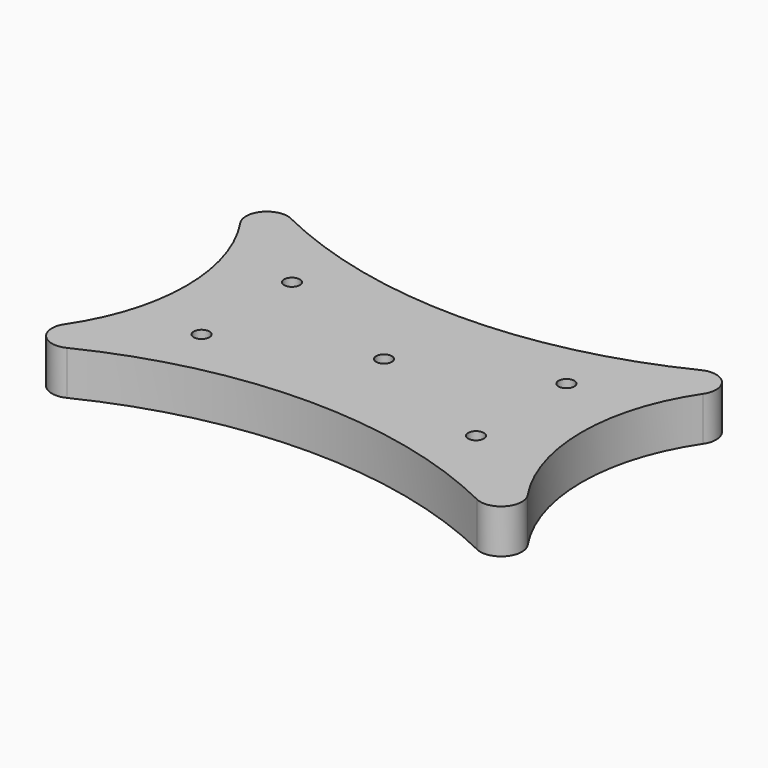
from build123d import *

# Parameters (mm, degrees)
F0_R     = 3.175
F1_DEPTH = 19.05
F2_DEPTH = 22.225
F3_DEPTH = 4.445


# Not quite as in the source:
# - a feature names something its author has since deleted; it is built from what else it names


with BuildPart() as f1:
    # F0 (on Top) → F1 (new body)
    with BuildSketch(Plane.XY):
        with BuildLine():
            ThreePointArc((82.8215071839, 56.5294814298), (0, 37.38), (-82.8215071839, 56.5294814298))
            ThreePointArc((-82.8215071839, 56.5294814298), (-92.8246316261, 54.4975844509), (-93.4439756283, 44.3089870526))
            ThreePointArc((-93.4439756283, 44.3089870526), (-79.88, 0), (-93.4439756283, -44.3089870526))
            ThreePointArc((-93.4439756283, -44.3089870526), (-92.8246316261, -54.4975844509), (-82.8215071839, -56.5294814298))
            ThreePointArc((-82.8215071839, -56.5294814298), (0, -37.38), (82.8215071839, -56.5294814298))
            ThreePointArc((82.8215071839, -56.5294814298), (92.8246316261, -54.4975844509), (93.4439756283, -44.3089870526))
            ThreePointArc((93.4439756283, -44.3089870526), (79.88, 0), (93.4439756283, 44.3089870526))
            ThreePointArc((93.4439756283, 44.3089870526), (92.8246316261, 54.4975844509), (82.8215071839, 56.5294814298))
        make_face()
        with Locations((-55.4007254541, -22.8000469506)):
            Circle(F0_R, mode=Mode.SUBTRACT)
        Circle(F0_R, mode=Mode.SUBTRACT)
        with Locations((55.4007254541, -22.8000469506)):
            Circle(F0_R, mode=Mode.SUBTRACT)
        with Locations((-55.4007254541, 22.8000469506)):
            Circle(F0_R, mode=Mode.SUBTRACT)
        with Locations((55.4007254541, 22.8000469506)):
            Circle(F0_R, mode=Mode.SUBTRACT)
    extrude(amount=F1_DEPTH)

    # F0 (on Top) → F2 (join)
    with BuildSketch(Plane.XY):
        with BuildLine():
            ThreePointArc((82.8215071839, 56.5294814298), (0, 37.38), (-82.8215071839, 56.5294814298))
            ThreePointArc((-82.8215071839, 56.5294814298), (-92.8246316261, 54.4975844509), (-93.4439756283, 44.3089870526))
            ThreePointArc((-93.4439756283, 44.3089870526), (-79.88, 0), (-93.4439756283, -44.3089870526))
            ThreePointArc((-93.4439756283, -44.3089870526), (-92.8246316261, -54.4975844509), (-82.8215071839, -56.5294814298))
            ThreePointArc((-82.8215071839, -56.5294814298), (0, -37.38), (82.8215071839, -56.5294814298))
            ThreePointArc((82.8215071839, -56.5294814298), (92.8246316261, -54.4975844509), (93.4439756283, -44.3089870526))
            ThreePointArc((93.4439756283, -44.3089870526), (79.88, 0), (93.4439756283, 44.3089870526))
            ThreePointArc((93.4439756283, 44.3089870526), (92.8246316261, 54.4975844509), (82.8215071839, 56.5294814298))
        make_face()
        with Locations((-55.4007254541, -22.8000469506)):
            Circle(F0_R, mode=Mode.SUBTRACT)
        Circle(F0_R, mode=Mode.SUBTRACT)
        with Locations((55.4007254541, -22.8000469506)):
            Circle(F0_R, mode=Mode.SUBTRACT)
        with Locations((-55.4007254541, 22.8000469506)):
            Circle(F0_R, mode=Mode.SUBTRACT)
        with Locations((55.4007254541, 22.8000469506)):
            Circle(F0_R, mode=Mode.SUBTRACT)
    extrude(amount=F2_DEPTH)

    # F0 (on Top) → F3 (cut)
    with BuildSketch(Plane.XY):
        with BuildLine():
            ThreePointArc((82.8215071839, 56.5294814298), (0, 37.38), (-82.8215071839, 56.5294814298))
            ThreePointArc((-82.8215071839, 56.5294814298), (-92.8246316261, 54.4975844509), (-93.4439756283, 44.3089870526))
            ThreePointArc((-93.4439756283, 44.3089870526), (-79.88, 0), (-93.4439756283, -44.3089870526))
            ThreePointArc((-93.4439756283, -44.3089870526), (-92.8246316261, -54.4975844509), (-82.8215071839, -56.5294814298))
            ThreePointArc((-82.8215071839, -56.5294814298), (0, -37.38), (82.8215071839, -56.5294814298))
            ThreePointArc((82.8215071839, -56.5294814298), (92.8246316261, -54.4975844509), (93.4439756283, -44.3089870526))
            ThreePointArc((93.4439756283, -44.3089870526), (79.88, 0), (93.4439756283, 44.3089870526))
            ThreePointArc((93.4439756283, 44.3089870526), (92.8246316261, 54.4975844509), (82.8215071839, 56.5294814298))
        make_face()
        with Locations((-55.4007254541, -22.8000469506)):
            Circle(F0_R, mode=Mode.SUBTRACT)
        Circle(F0_R, mode=Mode.SUBTRACT)
        with Locations((55.4007254541, -22.8000469506)):
            Circle(F0_R, mode=Mode.SUBTRACT)
        with Locations((-55.4007254541, 22.8000469506)):
            Circle(F0_R, mode=Mode.SUBTRACT)
        with Locations((55.4007254541, 22.8000469506)):
            Circle(F0_R, mode=Mode.SUBTRACT)
    extrude(amount=F3_DEPTH, mode=Mode.SUBTRACT)


solid = f1.part
